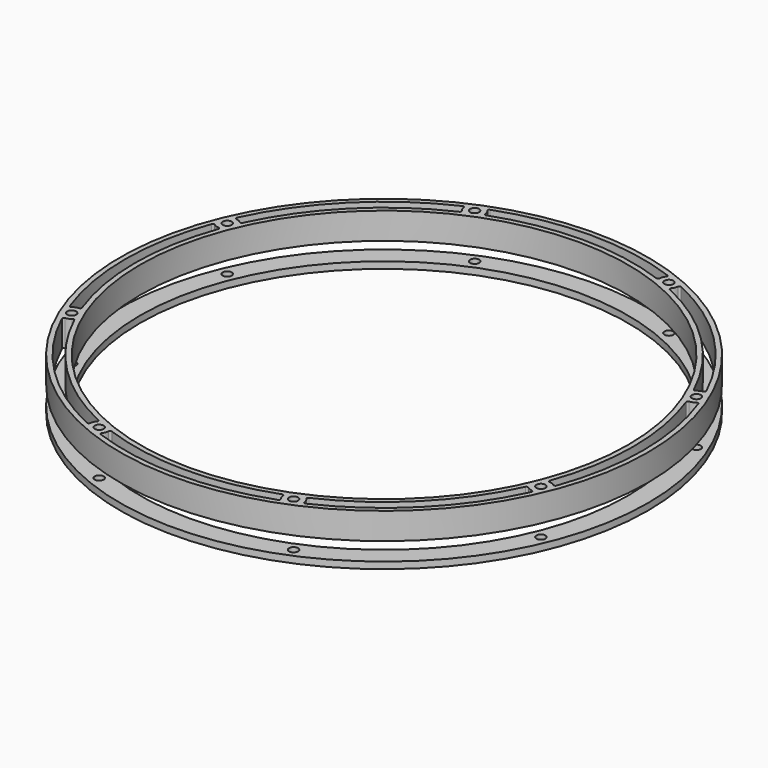
from build123d import *

# Parameters (mm, degrees)
F0_R            = 125.7624739
F0_R_2          = 2.15265
F0_R_3          = 116.2374739
F1_DEPTH        = 12.7
F3_DEPTH        = 12.7
F3_COPIES_COUNT = 8
F4_R            = 0.762
F7_R            = 125.7624739
F7_R_2          = 2.15265
F7_R_3          = 116.2374739
F8_DEPTH        = 1.5875


# Not quite as in the source:
# - a feature of the source that left no trace in its solid (it failed there, or was rolled back) is left out
# - a pattern or mirror of a feature is missing from the dataset's text; its kind, count and spacing are read off the source's solid


with BuildPart() as f1:
    # F0 (on Top) → F1 (new body)
    with BuildSketch(Plane.XY):
        Circle(F0_R)
        with Locations((-46.3046853281, -111.7893993206)):
            Circle(F0_R_2, mode=Mode.SUBTRACT)
        with Locations((-111.7893993206, -46.3046853281)):
            Circle(F0_R_2, mode=Mode.SUBTRACT)
        with Locations((46.3046853281, -111.7893993206)):
            Circle(F0_R_2, mode=Mode.SUBTRACT)
        with Locations((111.7893993206, -46.3046853281)):
            Circle(F0_R_2, mode=Mode.SUBTRACT)
        with Locations((-111.7893993206, 46.3046853281)):
            Circle(F0_R_2, mode=Mode.SUBTRACT)
        with Locations((-46.3046853281, 111.7893993206)):
            Circle(F0_R_2, mode=Mode.SUBTRACT)
        Circle(F0_R_3, mode=Mode.SUBTRACT)
        with Locations((111.7893993206, 46.3046853281)):
            Circle(F0_R_2, mode=Mode.SUBTRACT)
        with Locations((46.3046853281, 111.7893993206)):
            Circle(F0_R_2, mode=Mode.SUBTRACT)
    extrude(amount=F1_DEPTH)

    # F2 (on face) → F3 (cut, through all)
    with BuildSketch(Plane.XY.offset(12.7)):
        with BuildLine():
            ThreePointArc((-112.3308593172, 51.0363052751), (-109.8921410428, 50.6729592753), (-107.9619507449, 49.1387713625))
            ThreePointArc((-107.9619507449, 49.1387713625), (-83.8761040454, 83.8761040454), (-49.1387713625, 107.9619507449))
            ThreePointArc((-49.1387713625, 107.9619507449), (-50.6729592753, 109.8921410428), (-51.0363052751, 112.3308593172))
            ThreePointArc((-51.0363052751, 112.3308593172), (-87.2437000908, 87.2437000908), (-112.3308593172, 51.0363052751))
        make_face()
    f3 = extrude(amount=-F3_DEPTH, mode=Mode.SUBTRACT)

    # F3_copies: F3 ×8 about axis
    f3_copies_axis = Axis((0, 0, 0), (0, 0, 1))
    for i in range(1, F3_COPIES_COUNT):
        add(f3.rotate(f3_copies_axis, i * 360 / F3_COPIES_COUNT), mode=Mode.SUBTRACT)

    # F4
    f4_edges = [f1.edges().sort_by_distance(p)[0] for p in [
        (-49.138771, 107.961951, 6.35),
        (-51.036305, 112.330859, 6.35),
        (-107.961951, 49.138771, 6.35),
        (-112.330859, 51.036305, 6.35),
        (-51.036305, -112.330859, 6.35),
        (-49.138771, -107.961951, 6.35),
        (-112.330859, -51.036305, 6.35),
        (-107.961951, -49.138771, 6.35),
        (-115.51803, -43.341795, 6.35),
        (-111.086986, -41.594269, 6.35),
        (-115.51803, 43.341795, 6.35),
        (-111.086986, 41.594269, 6.35),
        (43.341795, -115.51803, 6.35),
        (41.594269, -111.086986, 6.35),
        (-43.341795, -115.51803, 6.35),
        (-41.594269, -111.086986, 6.35),
        (112.330859, -51.036305, 6.35),
        (107.961951, -49.138771, 6.35),
        (51.036305, -112.330859, 6.35),
        (49.138771, -107.961951, 6.35),
        (-43.341795, 115.51803, 6.35),
        (-41.594269, 111.086986, 6.35),
        (41.594269, 111.086986, 6.35),
        (43.341795, 115.51803, 6.35),
        (115.51803, 43.341795, 6.35),
        (111.086986, 41.594269, 6.35),
        (115.51803, -43.341795, 6.35),
        (111.086986, -41.594269, 6.35),
        (51.036305, 112.330859, 6.35),
        (49.138771, 107.961951, 6.35),
        (112.330859, 51.036305, 6.35),
        (107.961951, 49.138771, 6.35),
    ]]
    fillet(f4_edges, radius=F4_R)


with BuildPart() as f8:
    # F7 (on offset) → F8 (new body, symmetric)
    with BuildSketch(Plane.XY.offset(-10.16)):
        Circle(F7_R)
        with Locations((-46.3046853281, -111.7893993206)):
            Circle(F7_R_2, mode=Mode.SUBTRACT)
        with Locations((-111.7893993206, -46.3046853281)):
            Circle(F7_R_2, mode=Mode.SUBTRACT)
        with Locations((46.3046853281, -111.7893993206)):
            Circle(F7_R_2, mode=Mode.SUBTRACT)
        with Locations((111.7893993206, -46.3046853281)):
            Circle(F7_R_2, mode=Mode.SUBTRACT)
        with Locations((-111.7893993206, 46.3046853281)):
            Circle(F7_R_2, mode=Mode.SUBTRACT)
        with Locations((-46.3046853281, 111.7893993206)):
            Circle(F7_R_2, mode=Mode.SUBTRACT)
        Circle(F7_R_3, mode=Mode.SUBTRACT)
        with Locations((111.7893993206, 46.3046853281)):
            Circle(F7_R_2, mode=Mode.SUBTRACT)
        with Locations((46.3046853281, 111.7893993206)):
            Circle(F7_R_2, mode=Mode.SUBTRACT)
    extrude(amount=F8_DEPTH, both=True)


solid = Compound([f1.part, f8.part])
